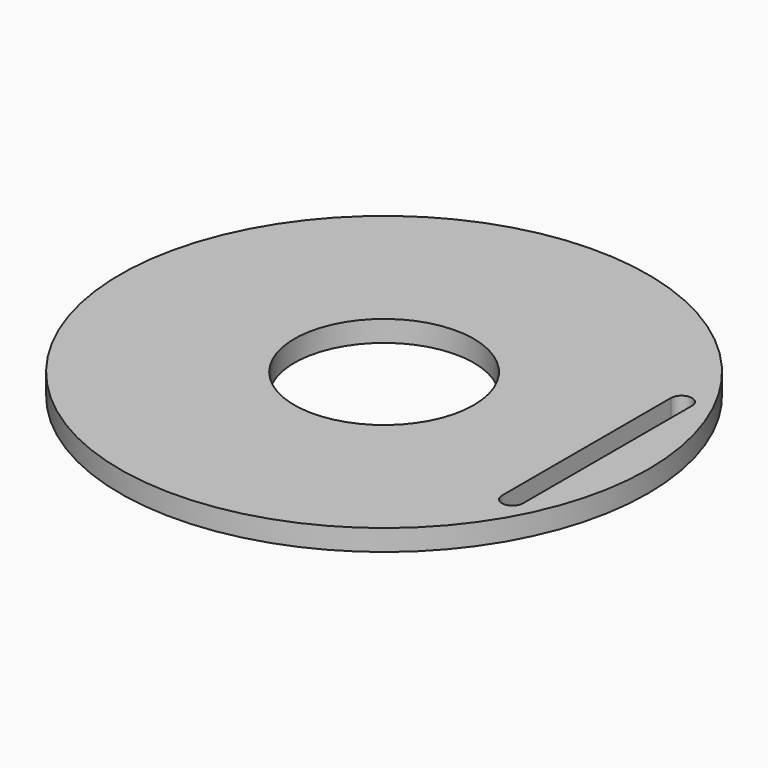
from build123d import *

# Parameters (mm, degrees)
F0_R     = 37.5
F0_R_2   = 12.75
F1_DEPTH = 3
F3_DEPTH = 3


# Not quite as in the source:
# - a feature names something its author has since deleted; it is built from what else it names


with BuildPart() as f1:
    # F0 (on Top) → F1 (new body)
    with BuildSketch(Plane.XY):
        Circle(F0_R)
        Circle(F0_R_2, mode=Mode.SUBTRACT)
    extrude(amount=F1_DEPTH)

    # F2 (on face) → F3 (cut, through all)
    with BuildSketch(Plane.XY.offset(3)):
        with BuildLine():
            Line((31.75, -15), (31.75, 15))
            ThreePointArc((31.75, 15), (30.25, 16.5), (28.75, 15))
            Line((28.75, 15), (28.75, -15))
            ThreePointArc((28.75, -15), (30.25, -16.5), (31.75, -15))
        make_face()
    extrude(amount=-F3_DEPTH, mode=Mode.SUBTRACT)


solid = f1.part
